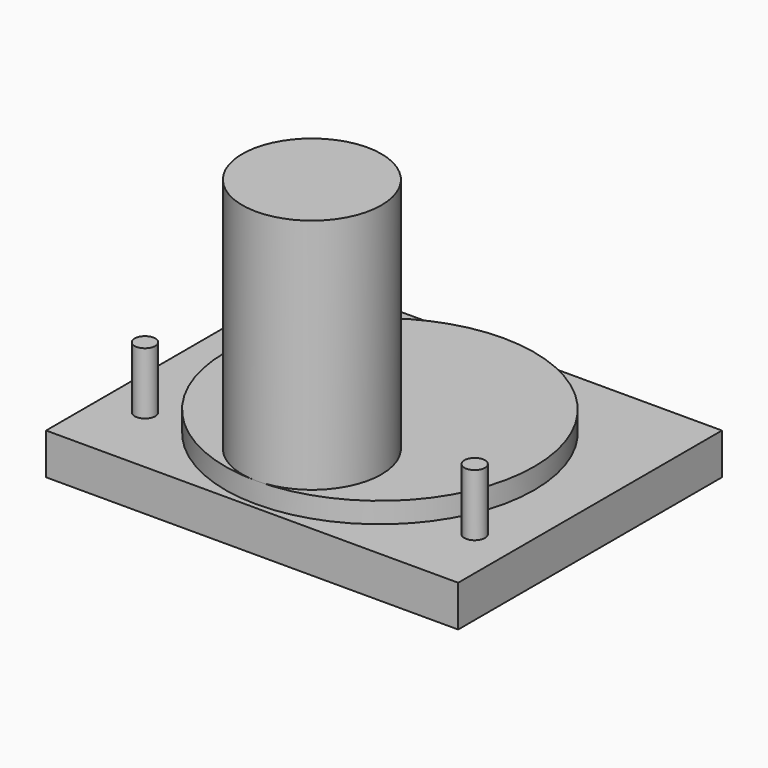
from build123d import *

# Parameters (mm, degrees)
F0_R     = 30
F1_DEPTH = 4
F3_DEPTH = 8
F4_R     = 2
F5_DEPTH = 12
F6_R     = 13.5
F7_DEPTH = 50


with BuildPart() as f1:
    # F0 (on Top) → F1 (new body)
    with BuildSketch(Plane.XY):
        Circle(F0_R)
    extrude(amount=-F1_DEPTH)

    # F2 (on face) → F3 (join)
    with BuildSketch(Plane(origin=(0, 0, -4), x_dir=(1, 0, 0), z_dir=(0, 0, -1))):
        Polygon((-40, 31), (-40, -33), (40, -33), (40, 31), (0, 31), align=None)
        with BuildLine():
            ThreePointArc((30, 0), (-21.2132034356, -21.2132034356), (0, 30))
            ThreePointArc((0, 30), (21.2132034356, 21.2132034356), (30, 0))
        make_face(mode=Mode.SUBTRACT)
        with BuildLine():
            ThreePointArc((30, 0), (21.2132034356, 21.2132034356), (0, 30))
            ThreePointArc((0, 30), (-21.2132034356, -21.2132034356), (30, 0))
        make_face()
    extrude(amount=F3_DEPTH)

    # F4 (on face) → F5 (join)
    with BuildSketch(Plane.XY.offset(-4)):
        with Locations((-32, -17)):
            Circle(F4_R)
        with Locations((32, -17)):
            Circle(F4_R)
    extrude(amount=F5_DEPTH)

    # F6 (on face) → F7 (join)
    with BuildSketch(Plane.XY.offset(-4)):
        with Locations((0, -16.5)):
            Circle(F6_R)
    extrude(amount=F7_DEPTH)


solid = f1.part
